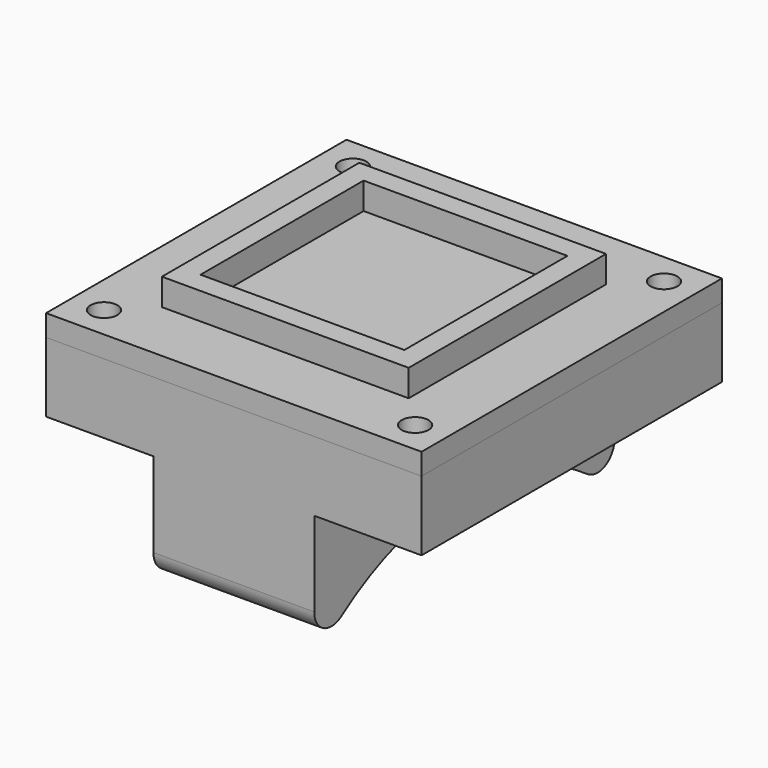
from build123d import *

# Parameters (mm, degrees)
F0_W       = 35
F0_H       = 35
F0_W_2     = 23
F0_H_2     = 23
F1_DEPTH   = 2
F3_DEPTH   = 5.5
F4_DEPTH   = 2.5
F5_DEPTH   = 1
F7_W       = 35
F7_H       = 35
F7_R       = 13.5
F8_DEPTH   = 1
F9_D       = 2.5
F9_DEPTH   = 10
F9_TIP     = 0.7510757738
F9_2_D     = 2.5
F9_2_DEPTH = 10
F9_2_TIP   = 0.7510757738
F10_W      = 7.5
F10_H      = 17.5
F11_DEPTH  = 25
F12_R      = 25
F13_DEPTH  = 25
F14_R      = 2


with BuildPart() as f1:
    # F0 (on Top) → F1 (new body)
    with BuildSketch(Plane.XY):
        with Locations((-9.5, 9.5)):
            Rectangle(F0_W, F0_H)
        with Locations((-9.5, 9.5)):
            Rectangle(F0_W_2, F0_H_2, mode=Mode.SUBTRACT)
        with Locations((-9.5, 9.5)):
            Rectangle(F0_W_2, F0_H_2)
        with BuildLine():
            Line((0, 5.027864045), (0, 0))
            Line((0, 0), (-5.027864045, 0))
            ThreePointArc((-5.027864045, 0), (-9.5, -1), (-13.972135955, 0))
            Line((-13.972135955, 0), (-19, 0))
            Line((-19, 0), (-19, 5.027864045))
            ThreePointArc((-19, 5.027864045), (-20, 9.5), (-19, 13.972135955))
            Line((-19, 13.972135955), (-19, 19))
            Line((-19, 19), (-13.972135955, 19))
            ThreePointArc((-13.972135955, 19), (-9.5, 20), (-5.027864045, 19))
            Line((-5.027864045, 19), (0, 19))
            Line((0, 19), (0, 13.972135955))
            ThreePointArc((0, 13.972135955), (0.746950766, 11.7912878475), (1, 9.5))
            ThreePointArc((1, 9.5), (0.746950766, 7.2087121525), (0, 5.027864045))
        make_face(mode=Mode.SUBTRACT)
        with BuildLine():
            Line((-13.972135955, 0), (-5.027864045, 0))
            ThreePointArc((-5.027864045, 0), (-2.0753787975, 2.0753787975), (0, 5.027864045))
            Line((0, 5.027864045), (0, 13.972135955))
            ThreePointArc((0, 13.972135955), (-2.0753787975, 16.9246212025), (-5.027864045, 19))
            Line((-5.027864045, 19), (-13.972135955, 19))
            ThreePointArc((-13.972135955, 19), (-16.9246212025, 16.9246212025), (-19, 13.972135955))
            Line((-19, 13.972135955), (-19, 5.027864045))
            ThreePointArc((-19, 5.027864045), (-16.9246212025, 2.0753787975), (-13.972135955, 0))
        make_face()
        with BuildLine():
            Line((-19, 19), (-19, 13.972135955))
            ThreePointArc((-19, 13.972135955), (-16.9246212025, 16.9246212025), (-13.972135955, 19))
            Line((-13.972135955, 19), (-19, 19))
        make_face()
        with BuildLine():
            ThreePointArc((-5.027864045, 19), (-2.0753787975, 16.9246212025), (0, 13.972135955))
            Line((0, 13.972135955), (0, 19))
            Line((0, 19), (-5.027864045, 19))
        make_face()
        with BuildLine():
            Line((-5.027864045, 0), (0, 0))
            Line((0, 0), (0, 5.027864045))
            ThreePointArc((0, 5.027864045), (-2.0753787975, 2.0753787975), (-5.027864045, 0))
        make_face()
        with BuildLine():
            Line((-19, 0), (-13.972135955, 0))
            ThreePointArc((-13.972135955, 0), (-16.9246212025, 2.0753787975), (-19, 5.027864045))
            Line((-19, 5.027864045), (-19, 0))
        make_face()
        with BuildLine():
            Line((0, 13.972135955), (0, 5.027864045))
            ThreePointArc((0, 5.027864045), (0.746950766, 7.2087121525), (1, 9.5))
            ThreePointArc((1, 9.5), (0.746950766, 11.7912878475), (0, 13.972135955))
        make_face()
        with BuildLine():
            ThreePointArc((-13.972135955, 0), (-9.5, -1), (-5.027864045, 0))
            Line((-5.027864045, 0), (-13.972135955, 0))
        make_face()
        with BuildLine():
            ThreePointArc((-19, 13.972135955), (-20, 9.5), (-19, 5.027864045))
            Line((-19, 5.027864045), (-19, 13.972135955))
        make_face()
        with BuildLine():
            Line((-13.972135955, 19), (-5.027864045, 19))
            ThreePointArc((-5.027864045, 19), (-9.5, 20), (-13.972135955, 19))
        make_face()
    extrude(amount=-F1_DEPTH)

    # F0 (on Top) → F4 (join)
    with BuildSketch(Plane.XY):
        with Locations((-9.5, 9.5)):
            Rectangle(F0_W_2, F0_H_2)
        with BuildLine():
            Line((0, 5.027864045), (0, 0))
            Line((0, 0), (-5.027864045, 0))
            ThreePointArc((-5.027864045, 0), (-9.5, -1), (-13.972135955, 0))
            Line((-13.972135955, 0), (-19, 0))
            Line((-19, 0), (-19, 5.027864045))
            ThreePointArc((-19, 5.027864045), (-20, 9.5), (-19, 13.972135955))
            Line((-19, 13.972135955), (-19, 19))
            Line((-19, 19), (-13.972135955, 19))
            ThreePointArc((-13.972135955, 19), (-9.5, 20), (-5.027864045, 19))
            Line((-5.027864045, 19), (0, 19))
            Line((0, 19), (0, 13.972135955))
            ThreePointArc((0, 13.972135955), (0.746950766, 11.7912878475), (1, 9.5))
            ThreePointArc((1, 9.5), (0.746950766, 7.2087121525), (0, 5.027864045))
        make_face(mode=Mode.SUBTRACT)
        with BuildLine():
            ThreePointArc((-19, 13.972135955), (-20, 9.5), (-19, 5.027864045))
            Line((-19, 5.027864045), (-19, 13.972135955))
        make_face()
        with BuildLine():
            Line((-13.972135955, 19), (-5.027864045, 19))
            ThreePointArc((-5.027864045, 19), (-9.5, 20), (-13.972135955, 19))
        make_face()
        with BuildLine():
            Line((0, 13.972135955), (0, 5.027864045))
            ThreePointArc((0, 5.027864045), (0.746950766, 7.2087121525), (1, 9.5))
            ThreePointArc((1, 9.5), (0.746950766, 11.7912878475), (0, 13.972135955))
        make_face()
        with BuildLine():
            ThreePointArc((-13.972135955, 0), (-9.5, -1), (-5.027864045, 0))
            Line((-5.027864045, 0), (-13.972135955, 0))
        make_face()
    extrude(amount=F4_DEPTH)


with BuildPart() as f3:
    # F2 (on face) → F3 (new body)
    with BuildSketch(Plane(origin=(0, 0, -2), x_dir=(1, 0, 0), z_dir=(0, 0, -1))):
        with BuildLine():
            Line((-27, -9.5), (-27, -27))
            Line((-27, -27), (8, -27))
            Line((8, -27), (8, -9.5))
            Line((8, -9.5), (4, -9.5))
            ThreePointArc((4, -9.5), (-9.5, -23), (-23, -9.5))
            Line((-23, -9.5), (-27, -9.5))
        make_face()
        with BuildLine():
            Line((-27, 8), (-27, -9.5))
            Line((-27, -9.5), (-23, -9.5))
            ThreePointArc((-23, -9.5), (-9.5, 4), (4, -9.5))
            Line((4, -9.5), (8, -9.5))
            Line((8, -9.5), (8, 8))
            Line((8, 8), (-27, 8))
        make_face()
    extrude(amount=F3_DEPTH)


with BuildPart() as f5:
    # F5 (new): a face of the model
    f5_faces = [f3.part.faces().sort_by_distance(p)[0] for p in [
        (-9.5, 26.5050252532, -7.5),
    ]]
    extrude(f5_faces, amount=F5_DEPTH)


with BuildPart() as f5b:
    # F5#2 (new): a face of the model
    f5_2_faces = [f1.part.faces().sort_by_distance(p)[0] for p in [
        (-9.5, 9.5, -2),
    ]]
    extrude(f5_2_faces, amount=F5_DEPTH)


with BuildPart() as f3_1:
    add(f3.part)

    # F7 (on face) → F8 (join)
    with BuildSketch(Plane(origin=(0, 0, -7.5), x_dir=(1, 0, 0), z_dir=(0, 0, -1))):
        with Locations((-9.5, -9.5)):
            Rectangle(F7_W, F7_H)
        with Locations((-9.5, -9.5)):
            Circle(F7_R, mode=Mode.SUBTRACT)
        with Locations((-9.5, -9.5)):
            Circle(F7_R)
    extrude(amount=F8_DEPTH)

    # F9#2
    with Locations(Plane.XY):
        with Locations((-24, -5), (-24, 24), (5, 24), (5, -5)):
            Hole(F9_2_D / 2, depth=F9_2_DEPTH)
            with Locations((0, 0, -(F9_2_DEPTH + F9_2_TIP / 2))):  # 118° drill point
                Cone(0, F9_2_D / 2, F9_2_TIP, mode=Mode.SUBTRACT)

    # F10 (on face) → F11 (join)
    with BuildSketch(Plane(origin=(0, 0, -8.5), x_dir=(1, 0, 0), z_dir=(0, 0, -1))):
        with Locations((-13.25, -0.75)):
            Rectangle(F10_W, F10_H)
        with Locations((-13.25, -18.25)):
            Rectangle(F10_W, F10_H)
        Polygon((-2, 8), (-9.5, 8), (-9.5, -9.5), (-9.5, -27), (-2, -27), (-2, -9.5), align=None)
    extrude(amount=F11_DEPTH)

    # F12 (on face) → F13 (cut)
    with BuildSketch(Plane(origin=(-17, 0, 0), x_dir=(0, -1, 0), z_dir=(-1, 0, 0))):
        with Locations((-9.5, -38.5)):
            Circle(F12_R)
    extrude(amount=-F13_DEPTH, mode=Mode.SUBTRACT)

    # F14
    f14_edges = [f3_1.edges().sort_by_distance(p)[0] for p in [
        (-9.5, -8, -20.646429),
        (-9.5, 27, -20.646429),
    ]]
    fillet(f14_edges, radius=F14_R)


with BuildPart() as f1_1:
    add(f1.part)

    # F9
    with Locations(Plane.XY):
        with Locations((-24, -5), (-24, 24), (5, 24), (5, -5)):
            Hole(F9_D / 2, depth=F9_DEPTH)
            with Locations((0, 0, -(F9_DEPTH + F9_TIP / 2))):  # 118° drill point
                Cone(0, F9_D / 2, F9_TIP, mode=Mode.SUBTRACT)


solid = Compound([f3_1.part, f1_1.part])
